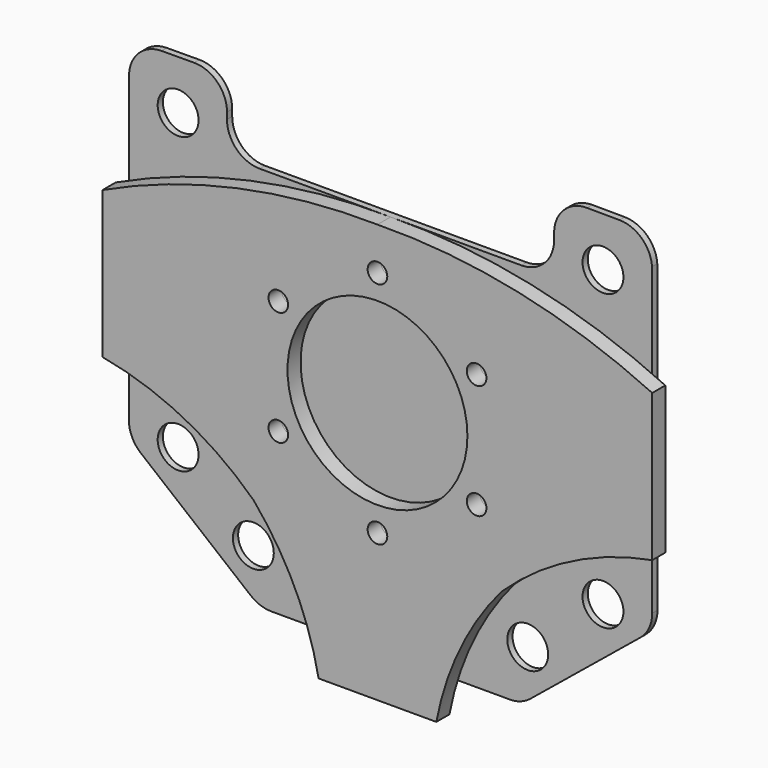
from build123d import *

# Parameters (mm, degrees)
F0_R     = 3
F1_DEPTH = 5
F2_R     = 6.25
F2_R_2   = 3
F3_DEPTH = 2


# Not quite as in the source:
# - a feature names something its author has since deleted; it is built from what else it names


with BuildPart() as f1:
    # F0 (on Front) → F1 (new body)
    with BuildSketch(Plane.XZ):
        with BuildLine():
            ThreePointArc((18, -80), (25.2450835608, -57.9435000854), (37.8911830779, -38.474124356))
            ThreePointArc((37.8911830779, -38.474124356), (59.2223421632, -23.3521866114), (84, -15))
            Line((84, -15), (84, 30))
            ThreePointArc((84, 30), (43.0306603199, 43.8097481595), (0, 48))
            ThreePointArc((0, 48), (-43.0306603199, 43.8097481595), (-84, 30))
            Line((-84, 30), (-84, -15))
            ThreePointArc((-84, -15), (-59.2223421632, -23.3521866114), (-37.8911830779, -38.474124356))
            ThreePointArc((-37.8911830779, -38.474124356), (-25.2450835608, -57.9435000854), (-18, -80))
            Line((-18, -80), (0, -80))
            Line((0, -80), (18, -80))
        make_face()
        with Locations((-30.3108891325, -17.5)):
            Circle(F0_R, mode=Mode.SUBTRACT)
        with Locations((0, -35)):
            Circle(F0_R, mode=Mode.SUBTRACT)
        with Locations((30.3108891325, -17.5)):
            Circle(F0_R, mode=Mode.SUBTRACT)
        with Locations((-30.3108891325, 17.5)):
            Circle(F0_R, mode=Mode.SUBTRACT)
        with BuildLine():
            ThreePointArc((19.2964358267, -19.5933040702), (-25.3663358138, 10.6206877076), (27.5, 0))
            ThreePointArc((27.5, 0), (25.3663358138, -10.6206877076), (19.2964358267, -19.5933040702))
        make_face(mode=Mode.SUBTRACT)
        with Locations((30.3108891325, 17.5)):
            Circle(F0_R, mode=Mode.SUBTRACT)
        with Locations((0, 35)):
            Circle(F0_R, mode=Mode.SUBTRACT)
    extrude(amount=F1_DEPTH)


with BuildPart() as f3:
    # F2 (on Front) → F3 (new body)
    with BuildSketch(Plane.XZ):
        with BuildLine():
            Line((40, 48), (0, 48))
            Line((0, 48), (-40, 48))
            ThreePointArc((-40, 48), (-47.0710678119, 50.9289321881), (-50, 58))
            Line((-50, 58), (-50, 60.0001774362))
            ThreePointArc((-50, 60.0001774362), (-52.9500251451, 67.0922754718), (-60.0595709092, 70))
            Line((-60.0595709092, 70), (-70.0243862443, 69.9406376358))
            ThreePointArc((-70.0243862443, 69.9406376358), (-76.8142082584, 67.2268164845), (-79.9418990419, 60.6174247888))
            Line((-79.9418990419, 60.6174247888), (-79.9971823925, -32.6300462499))
            ThreePointArc((-79.9971823925, -32.6300462499), (-79.0316227544, -36.923039078), (-76.3168067264, -40.3859665636))
            Line((-76.3168067264, -40.3859665636), (-42.7592701532, -67.7499916446))
            ThreePointArc((-42.7592701532, -67.7499916446), (-39.7937557707, -69.4207196234), (-36.4396475767, -70))
            Line((-36.4396475767, -70), (0, -70))
            Line((0, -70), (36.4396475767, -70))
            ThreePointArc((36.4396475767, -70), (39.7937557707, -69.4207196234), (42.7592701532, -67.7499916446))
            Line((42.7592701532, -67.7499916446), (76.3168067264, -40.3859665636))
            ThreePointArc((76.3168067264, -40.3859665636), (79.0316227544, -36.923039078), (79.9971823925, -32.6300462499))
            Line((79.9971823925, -32.6300462499), (79.9418990419, 60.6174247888))
            ThreePointArc((79.9418990419, 60.6174247888), (76.8142082584, 67.2268164845), (70.0243862443, 69.9406376358))
            Line((70.0243862443, 69.9406376358), (60.0595709092, 70))
            ThreePointArc((60.0595709092, 70), (52.9500251451, 67.0922754718), (50, 60.0001774362))
            Line((50, 60.0001774362), (50, 58))
            ThreePointArc((50, 58), (47.0710678119, 50.9289321881), (40, 48))
        make_face()
        with Locations((-41.9418990419, -54.0593623642)):
            Circle(F2_R, mode=Mode.SUBTRACT)
        with Locations((-64.9418990419, -35.0593623642)):
            Circle(F2_R, mode=Mode.SUBTRACT)
        with Locations((-30.3108891325, -17.5)):
            Circle(F2_R_2, mode=Mode.SUBTRACT)
        with Locations((0, -35)):
            Circle(F2_R_2, mode=Mode.SUBTRACT)
        with Locations((41.9418990419, -54.0593623642)):
            Circle(F2_R, mode=Mode.SUBTRACT)
        with Locations((64.9418990419, -35.0593623642)):
            Circle(F2_R, mode=Mode.SUBTRACT)
        with Locations((30.3108891325, -17.5)):
            Circle(F2_R_2, mode=Mode.SUBTRACT)
        with Locations((-30.3108891325, 17.5)):
            Circle(F2_R_2, mode=Mode.SUBTRACT)
        with Locations((-64.9418990419, 54.9406376358)):
            Circle(F2_R, mode=Mode.SUBTRACT)
        with Locations((30.3108891325, 17.5)):
            Circle(F2_R_2, mode=Mode.SUBTRACT)
        with BuildLine():
            ThreePointArc((0, 32), (-3, 35), (0, 38))
            ThreePointArc((0, 38), (2.1213203436, 37.1213203436), (3, 35))
            ThreePointArc((3, 35), (2.1213203436, 32.8786796564), (0, 32))
        make_face(mode=Mode.SUBTRACT)
        with Locations((64.9418990419, 54.9406376358)):
            Circle(F2_R, mode=Mode.SUBTRACT)
    extrude(amount=-F3_DEPTH)


solid = Compound([f1.part, f3.part])
